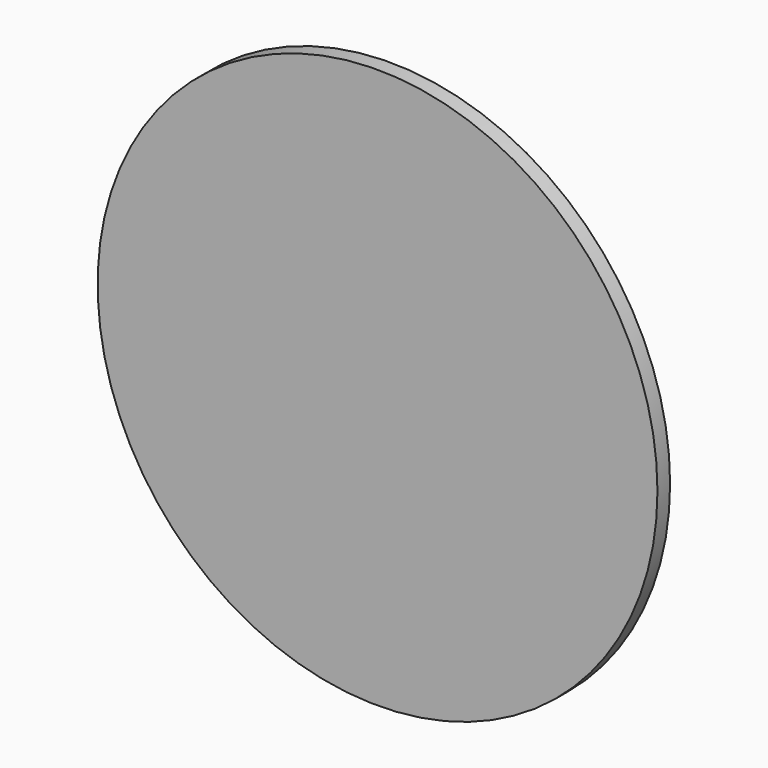
from build123d import *

# Parameters (mm, degrees)
F0_R         = 45.0347180744
F1_DEPTH     = 2.54
F2_TEXT_SIZE = 20.7254022826
F3_DEPTH     = 0.254


# Not quite as in the source:
# - Text() gives the source's letters only with a copy of the font that has no kerning and outlines rounded to 1/6400 em; it was checked with that copy


with BuildPart() as f1:
    # F0 (on Front) → F1 (new body)
    with BuildSketch(Plane.XZ):
        Circle(F0_R)
    extrude(amount=F1_DEPTH)

    # F2 (on face) → F3 (join)
    with BuildSketch(Plane(origin=(0, 0, 0), x_dir=(-1, 0, 0), z_dir=(0, 1, 0))):
        with Locations((-27.269449085, -5.7483534329)):
            Text('Mom', F2_TEXT_SIZE, font='Open Sans', text_align=(TextAlign.LEFT, TextAlign.BOTTOM))
    extrude(amount=F3_DEPTH)


solid = f1.part
